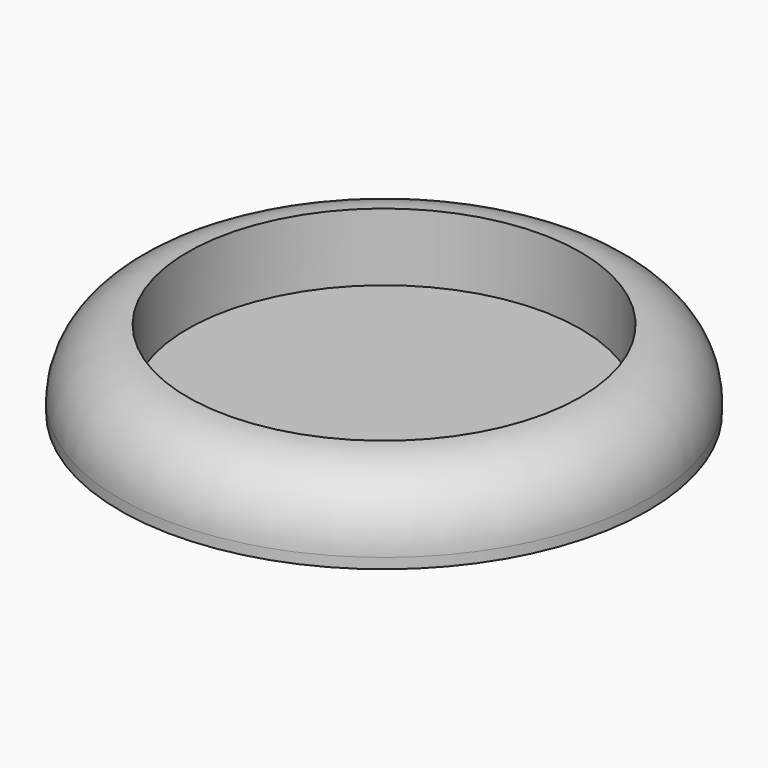
from build123d import *

# Parameters (mm, degrees)
F0_R     = 50.8
F0_R_2   = 37.8
F1_DEPTH = 2
F2_DEPTH = 13
F3_R     = 12.99999


# Not quite as in the source:
# - a fillet or chamfer is up to 0.001 mm smaller than in the source, because OpenCascade refuses the exact size


with BuildPart() as f1:
    # F0 (on Top) → F1 (new body)
    with BuildSketch(Plane.XY):
        Circle(F0_R)
        Circle(F0_R_2, mode=Mode.SUBTRACT)
        Circle(F0_R_2)
    extrude(amount=-F1_DEPTH)

    # F0 (on Top) → F2 (join)
    with BuildSketch(Plane.XY):
        Circle(F0_R)
        Circle(F0_R_2, mode=Mode.SUBTRACT)
    extrude(amount=F2_DEPTH)

    # F3 (radius 13 in the source; OpenCascade refuses exactly that, so slightly less here)
    f3_edges = [f1.edges().sort_by_distance(p)[0] for p in [
        (-50.8, 0, 13),
    ]]
    fillet(f3_edges, radius=F3_R)


solid = f1.part
